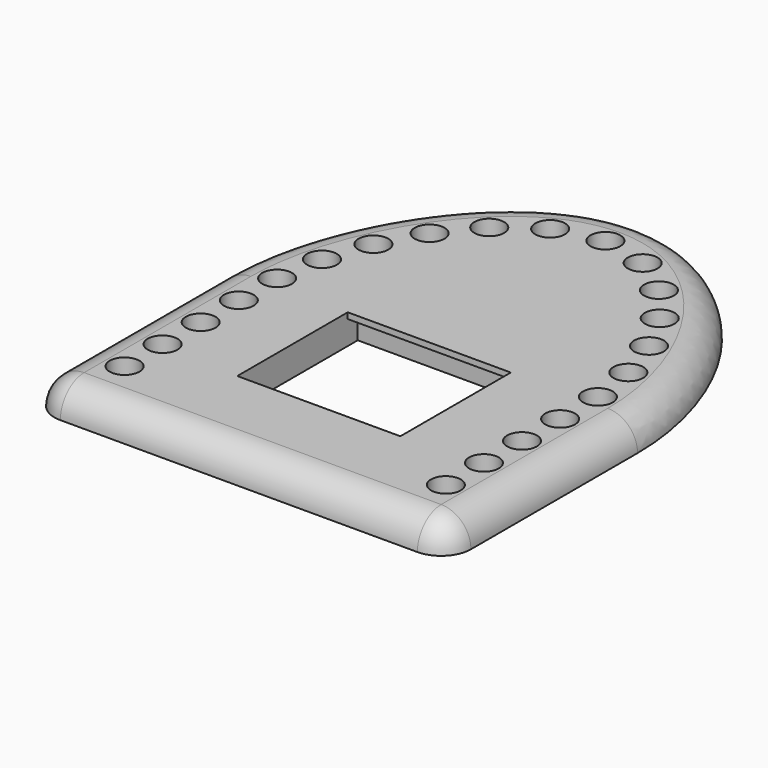
from build123d import *

# Parameters (mm, degrees)
F0_W     = 27.4
F0_H     = 2.1
F1_DEPTH = 5
F2_DEPTH = 4
F3_D     = 5
F4_R     = 4.9999


# Not quite as in the source:
# - a fillet or chamfer is up to 0.001 mm smaller than in the source, because OpenCascade refuses the exact size
# - ends of sketch curves that miss each other by under 0.0002 mm in the source are joined
# - a feature names something its author has since deleted; it is built from what else it names


with BuildPart() as f1:
    # F0 (on Top) → F1 (new body)
    with BuildSketch(Plane.XY):
        with BuildLine():
            Line((-35, 2.1762e-06), (-35, -40))
            Line((-35, -40), (-27, -40))
            Line((-27, -40), (-27, -22.2710574513))
            ThreePointArc((-27, -22.2710574513), (-32.9393385518, -11.8321585422), (-35, 2.1762e-06))
        make_face()
        with BuildLine():
            Line((-27, -22.2710574513), (-27, -40))
            Line((-27, -40), (27, -40))
            Line((27, -40), (27, -22.2710574513))
            ThreePointArc((27, -22.2710574513), (0, -35), (-27, -22.2710574513))
        make_face()
        with BuildLine():
            add(Edge.make_bspline(
                [(0, 45), (-20.1986748725, 45), (-35, 20.0504870868), (-35, 2.1762e-06)],
                knots=[0, 0, 0, 0, 57.0087695372, 57.0087695372, 57.0087695372, 57.0087695372], degree=3))
            ThreePointArc((-35, 2.1762e-06), (-28.4666369261, 20.3629708568), (-11.3056830814, 33.1237306181))
            add(Edge.make_bspline(
                [(0, 37), (-0.2833414452, 37.0069688983), (-1.1232932293, 37.0068386903), (-2.7957299856, 36.8864035146), (-4.9942322029, 36.3521195303), (-7.6997383876, 35.2871018647), (-9.7958540485, 34.148638444), (-11.0540635502, 33.3003360386), (-11.3056830814, 33.1237306181)],
                knots=[0, 0, 0, 0, 0.8506820357, 2.5185967411, 5.0181648841, 7.6012051941, 11.2266191262, 12.1476935207, 12.1476935207, 12.1476935207, 12.1476935207], degree=3))
            add(Edge.make_bspline(
                [(0, 37), (0.2833414452, 37.0069688983), (1.1232932293, 37.0068386903), (2.7957299856, 36.8864035146), (4.9942322029, 36.3521195303), (7.6997383876, 35.2871018647), (9.7958540485, 34.148638444), (11.0540635502, 33.3003360386), (11.3056830814, 33.1237306181)],
                knots=[0, 0, 0, 0, 0.8506820357, 2.5185967411, 5.0181648841, 7.6012051941, 11.2266191262, 12.1476935207, 12.1476935207, 12.1476935207, 12.1476935207], degree=3))
            ThreePointArc((11.3056830814, 33.1237306181), (28.4666375592, 20.3629699719), (35, 0))
            add(Edge.make_bspline(
                [(0, 45), (20.1986748725, 45), (35, 20.0504870868), (35, 0)],
                knots=[0, 0, 0, 0, 57.0087695372, 57.0087695372, 57.0087695372, 57.0087695372], degree=3))
        make_face()
        with BuildLine():
            ThreePointArc((-11.3056830814, 33.1237306181), (-28.4666369261, 20.3629708568), (-35, 2.1762e-06))
            ThreePointArc((-35, 2.1762e-06), (-32.9393385518, -11.8321585422), (-27, -22.2710574513))
            Line((-27, -22.2710574513), (-27, 2.1762e-06))
            add(Edge.make_bspline(
                [(-11.3056830814, 33.1237306181), (-12.4097508436, 32.3488132243), (-15.1414824386, 30.0752135158), (-18.8876274503, 25.5283101279), (-22.422035633, 19.604279738), (-25.0662594291, 13.1120426553), (-26.6478130576, 7.1844788974), (-27.0173066601, 2.7756083867), (-27.018694794, 0.6711028041), (-27, 2.1762e-06)],
                knots=[12.1476935207, 12.1476935207, 12.1476935207, 12.1476935207, 16.189226149, 22.7543847852, 29.7183326598, 36.8091409701, 43.7289829573, 48.0262708445, 50.0404462243, 50.0404462243, 50.0404462243, 50.0404462243], degree=3))
        make_face()
        with BuildLine():
            Line((27, -22.2710574513), (27, -40))
            Line((27, -40), (35, -40))
            Line((35, -40), (35, 0))
            ThreePointArc((35, 0), (32.939338184, -11.8321595662), (27, -22.2710574513))
        make_face()
        with BuildLine():
            Line((27, 2.1762e-06), (27, -22.2710574513))
            ThreePointArc((27, -22.2710574513), (32.939338184, -11.8321595662), (35, 0))
            ThreePointArc((35, 0), (28.4666375592, 20.3629699719), (11.3056830814, 33.1237306181))
            add(Edge.make_bspline(
                [(11.3056830814, 33.1237306181), (12.4097508436, 32.3488132243), (15.1414824386, 30.0752135158), (18.8876274503, 25.5283101279), (22.422035633, 19.604279738), (25.0662594291, 13.1120426553), (26.6478130576, 7.1844788974), (27.0173066601, 2.7756083867), (27.018694794, 0.6711028041), (27, 2.1762e-06)],
                knots=[12.1476935207, 12.1476935207, 12.1476935207, 12.1476935207, 16.189226149, 22.7543847852, 29.7183326598, 36.8091409701, 43.7289829573, 48.0262708445, 50.0404462243, 50.0404462243, 50.0404462243, 50.0404462243], degree=3))
        make_face()
        with BuildLine():
            add(Edge.make_bspline(
                [(0, 37), (-0.2833414452, 37.0069688983), (-1.1232932293, 37.0068386903), (-2.7957299856, 36.8864035146), (-4.9942322029, 36.3521195303), (-7.6997383876, 35.2871018647), (-9.7958540485, 34.148638444), (-11.0540635502, 33.3003360386), (-11.3056830814, 33.1237306181)],
                knots=[0, 0, 0, 0, 0.8506820357, 2.5185967411, 5.0181648841, 7.6012051941, 11.2266191262, 12.1476935207, 12.1476935207, 12.1476935207, 12.1476935207], degree=3))
            ThreePointArc((-11.3056830814, 33.1237306181), (0, 35), (11.3056830814, 33.1237306181))
            add(Edge.make_bspline(
                [(0, 37), (0.2833414452, 37.0069688983), (1.1232932293, 37.0068386903), (2.7957299856, 36.8864035146), (4.9942322029, 36.3521195303), (7.6997383876, 35.2871018647), (9.7958540485, 34.148638444), (11.0540635502, 33.3003360386), (11.3056830814, 33.1237306181)],
                knots=[0, 0, 0, 0, 0.8506820357, 2.5185967411, 5.0181648841, 7.6012051941, 11.2266191262, 12.1476935207, 12.1476935207, 12.1476935207, 12.1476935207], degree=3))
        make_face()
        with BuildLine():
            Line((-27, 2.1762e-06), (-27, -22.2710574513))
            ThreePointArc((-27, -22.2710574513), (0, -35), (27, -22.2710574513))
            Line((27, -22.2710574513), (27, 2.1762e-06))
            add(Edge.make_bspline(
                [(11.3056830814, 33.1237306181), (12.4097508436, 32.3488132243), (15.1414824386, 30.0752135158), (18.8876274503, 25.5283101279), (22.422035633, 19.604279738), (25.0662594291, 13.1120426553), (26.6478130576, 7.1844788974), (27.0173066601, 2.7756083867), (27.018694794, 0.6711028041), (27, 2.1762e-06)],
                knots=[12.1476935207, 12.1476935207, 12.1476935207, 12.1476935207, 16.189226149, 22.7543847852, 29.7183326598, 36.8091409701, 43.7289829573, 48.0262708445, 50.0404462243, 50.0404462243, 50.0404462243, 50.0404462243], degree=3))
            ThreePointArc((11.3056830814, 33.1237306181), (0, 35), (-11.3056830814, 33.1237306181))
            add(Edge.make_bspline(
                [(-11.3056830814, 33.1237306181), (-12.4097508436, 32.3488132243), (-15.1414824386, 30.0752135158), (-18.8876274503, 25.5283101279), (-22.422035633, 19.604279738), (-25.0662594291, 13.1120426553), (-26.6478130576, 7.1844788974), (-27.0173066601, 2.7756083867), (-27.018694794, 0.6711028041), (-27, 2.1762e-06)],
                knots=[12.1476935207, 12.1476935207, 12.1476935207, 12.1476935207, 16.189226149, 22.7543847852, 29.7183326598, 36.8091409701, 43.7289829573, 48.0262708445, 50.0404462243, 50.0404462243, 50.0404462243, 50.0404462243], degree=3))
        make_face()
        Polygon((-13.7, -23.2), (-13.7, 0), (-13.7, 2.1), (13.7, 2.1), (13.7, 0), (13.7, -23.2), (13.7, -25.3), (-13.7, -25.3), align=None, mode=Mode.SUBTRACT)
        with Locations((0, 1.05)):
            Rectangle(F0_W, F0_H)
        with Locations((0, -24.25)):
            Rectangle(F0_W, F0_H)
    extrude(amount=F1_DEPTH)

    # F0 (on Top) → F2 (cut)
    with BuildSketch(Plane.XY):
        with Locations((0, 1.05)):
            Rectangle(F0_W, F0_H)
        with Locations((0, -24.25)):
            Rectangle(F0_W, F0_H)
    extrude(amount=F2_DEPTH, mode=Mode.SUBTRACT)

    # F3 (through all)
    with Locations(Plane(origin=(0, 0, 0), x_dir=(1, 0, 0), z_dir=(0, 0, -1))):
        with Locations((0, -37), (-7.7739062126, -35.111513252), (-14.2579257305, -30.4256311694), (-19.3371352018, -24.244884358), (-23.1543015859, -17.2142911543), (-25.7431047524, -9.6447404302), (-26.9552512695, -1.7371048277), (-27, 6.2627700182), (-27, 14.2627700182), (-27, 22.2627700182), (7.7739062126, -35.111513252), (14.2579257305, -30.4256311694), (19.3371352018, -24.244884358), (23.1543015859, -17.2142911543), (25.7431047524, -9.6447404302), (26.9552512695, -1.7371048277), (27, 6.2627700182), (27, 14.2627700182), (27, 22.2627700182), (-27, 30.2627700182), (27, 30.2627700182)):
            Hole(F3_D / 2)

    # F4 (radius 5 in the source; OpenCascade refuses exactly that, so slightly less here)
    f4_edges = [f1.edges().sort_by_distance(p)[0] for p in [
        (-35, -40, 2.5),
        (35, -40, 2.5),
        (-35, -19.999999, 5),
        (0, -40, 5),
    ]]
    fillet(f4_edges, radius=F4_R)


solid = f1.part
